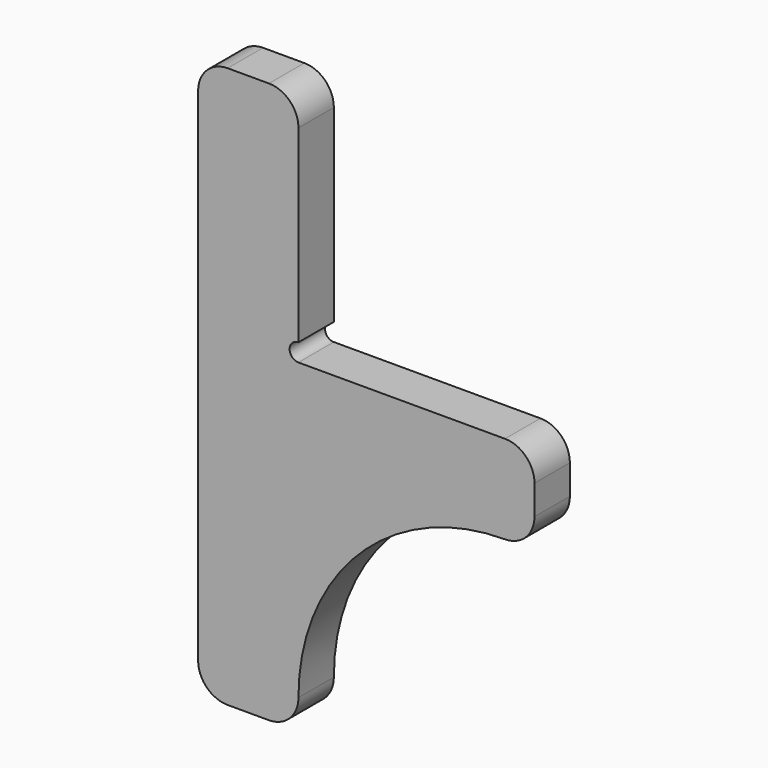
from build123d import *

# Parameters (mm, degrees)
F1_DEPTH = 19.05
F2_R     = 88.9
F3_R     = 12.69999
F5_DEPTH = 19.051


# Not quite as in the source:
# - a fillet or chamfer is up to 0.001 mm smaller than in the source, because OpenCascade refuses the exact size


with BuildPart() as f1:
    # F0 (on Front) → F1 (new body)
    with BuildSketch(Plane.XZ):
        Polygon((0, 241.3), (0, 0), (43.18, 0), (43.18, 101.6), (144.78, 101.6), (144.78, 139.7), (43.18, 139.7), (43.18, 241.3), align=None)
    extrude(amount=F1_DEPTH)

    # F2
    f2_edges = [f1.edges().sort_by_distance(p)[0] for p in [
        (43.18, -9.525, 101.6),
    ]]
    fillet(f2_edges, radius=F2_R)

    # F3 (radius 12.7 in the source; OpenCascade refuses exactly that, so slightly less here)
    f3_edges = [f1.edges().sort_by_distance(p)[0] for p in [
        (144.78, -9.525, 139.7),
        (144.78, -9.525, 101.6),
        (43.18, -9.525, 0),
        (43.18, -9.525, 241.3),
        (0, -9.525, 0),
        (0, -9.525, 241.3),
    ]]
    fillet(f3_edges, radius=F3_R)

    # F4 (on face) → F5 (cut, through all)
    with BuildSketch(Plane.XZ.offset(19.05)):
        with BuildLine():
            Line((43.18, 139.7), (43.18, 147.32))
            ThreePointArc((43.18, 147.32), (39.37, 143.51), (43.18, 139.7))
        make_face()
    extrude(amount=-F5_DEPTH, mode=Mode.SUBTRACT)


solid = f1.part
